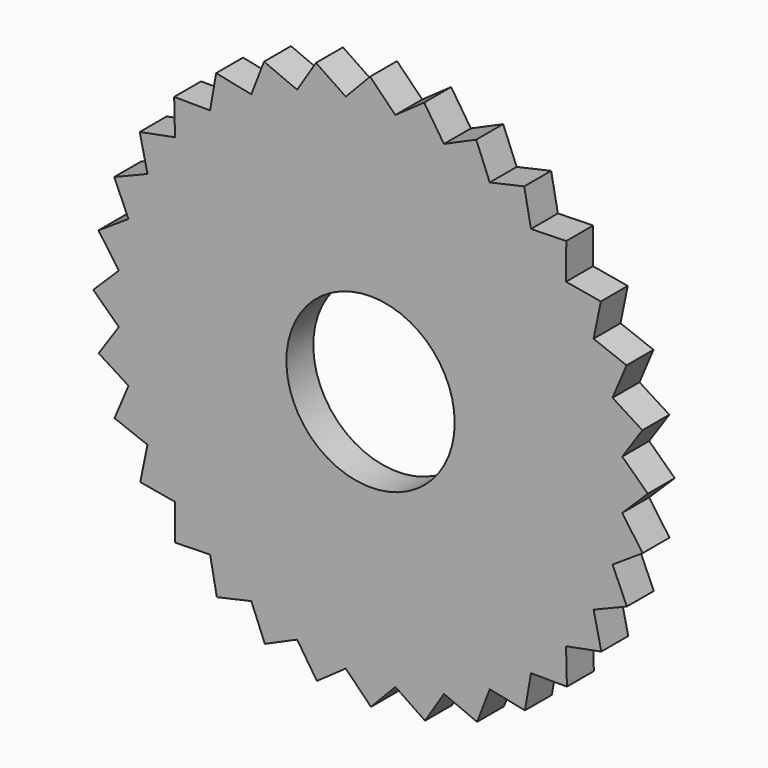
from build123d import *

# Parameters (mm, degrees)
F1_DEPTH = 5.08
F2_DEPTH = 5.08
F3_DEPTH = 5.08


with BuildPart() as f1:
    # F0 (on Front) → F1 (new body, symmetric)
    with BuildSketch(Plane.XZ):
        with BuildLine():
            ThreePointArc((75.8478085303, 7.3177825298), (76.1119012048, 3.6631263964), (76.2, 0))
            ThreePointArc((76.2, 0), (76.1119012048, -3.6631263964), (75.8478085303, -7.3177825298))
            Line((75.8478085303, -7.3177825298), (75.9612060886, -7.4788283967))
            Line((75.9612060886, -7.4788283967), (83.6803820326, 0.1329535853))
            Line((83.6803820326, 0.1329535853), (75.9606798536, 7.4841713504))
            Line((75.9606798536, 7.4841713504), (75.8478085303, 7.3177825298))
        make_face()
        with BuildLine():
            ThreePointArc((75.8180427075, 7.62), (75.8330761724, 7.4689060931), (75.8478085303, 7.3177825298))
            Line((75.8478085303, 7.3177825298), (75.9606798536, 7.4841713504))
            Line((75.9606798536, 7.4841713504), (75.8180427075, 7.62))
        make_face()
        with BuildLine():
            Line((75.9612060886, -7.4788283967), (75.8478085303, -7.3177825298))
            ThreePointArc((75.8478085303, -7.3177825298), (75.8330761724, -7.4689060931), (75.8180427075, -7.62))
            Line((75.8180427075, -7.62), (75.9612060886, -7.4788283967))
        make_face()
        with BuildLine():
            ThreePointArc((72.9627856072, 21.9743467808), (74.7358383667, 14.8658825376), (75.8180427075, 7.62))
            Line((75.8180427075, 7.62), (75.9606798536, 7.4841713504))
            Line((75.9606798536, 7.4841713504), (82.0465489983, 16.4556315966))
            Line((82.0465489983, 16.4556315966), (73.041027291, 22.1595585897))
            Line((73.041027291, 22.1595585897), (72.9627856072, 21.9743467808))
        make_face()
        with BuildLine():
            Line((75.9612060886, -7.4788283967), (75.8180427075, -7.62))
            ThreePointArc((75.8180427075, -7.62), (74.7358383667, -14.8658825376), (72.9627856072, -21.9743467808))
            Line((72.9627856072, -21.9743467808), (73.0425857732, -22.1544209627))
            Line((73.0425857732, -22.1544209627), (82.0984249139, -16.1948337577))
            Line((82.0984249139, -16.1948337577), (75.9612060886, -7.4788283967))
        make_face()
        with BuildLine():
            ThreePointArc((72.8746320228, 22.2649502031), (72.9188535828, 22.1196924068), (72.9627856072, 21.9743467808))
            Line((72.9627856072, 21.9743467808), (73.041027291, 22.1595585897))
            Line((73.041027291, 22.1595585897), (72.8746320228, 22.2649502031))
        make_face()
        with BuildLine():
            Line((73.0425857732, -22.1544209627), (72.9627856072, -21.9743467808))
            ThreePointArc((72.9627856072, -21.9743467808), (72.9188535828, -22.1196924068), (72.8746320228, -22.2649502031))
            Line((72.8746320228, -22.2649502031), (73.0425857732, -22.1544209627))
        make_face()
        with BuildLine():
            ThreePointArc((67.2738437512, 35.7864492084), (70.3996203774, 29.1604775462), (72.8746320228, 22.2649502031))
            Line((72.8746320228, 22.2649502031), (73.041027291, 22.1595585897))
            Line((73.041027291, 22.1595585897), (77.2597130983, 32.1459289141))
            Line((77.2597130983, 32.1459289141), (67.3144490116, 35.9833664196))
            Line((67.3144490116, 35.9833664196), (67.2738437512, 35.7864492084))
        make_face()
        with BuildLine():
            Line((73.0425857732, -22.1544209627), (72.8746320228, -22.2649502031))
            ThreePointArc((72.8746320228, -22.2649502031), (70.3996203774, -29.1604775462), (67.2738437512, -35.7864492084))
            Line((67.2738437512, -35.7864492084), (67.3169798492, -35.9786315554))
            Line((67.3169798492, -35.9786315554), (77.361471367, -31.9002627216))
            Line((77.361471367, -31.9002627216), (73.0425857732, -22.1544209627))
        make_face()
        with BuildLine():
            ThreePointArc((67.1306900979, 36.0542708563), (67.2024003433, 35.9204313461), (67.2738437512, 35.7864492084))
            Line((67.2738437512, 35.7864492084), (67.3144490116, 35.9833664196))
            Line((67.3144490116, 35.9833664196), (67.1306900979, 36.0542708563))
        make_face()
        with BuildLine():
            Line((67.3169798492, -35.9786315554), (67.2738437512, -35.7864492084))
            ThreePointArc((67.2738437512, -35.7864492084), (67.2024003433, -35.9204313461), (67.1306900979, -36.0542708563))
            Line((67.1306900979, -36.0542708563), (67.3169798492, -35.9786315554))
        make_face()
        with BuildLine():
            ThreePointArc((58.9996058074, 48.2232984621), (63.3579844575, 42.3344517561), (67.1306900979, 36.0542708563))
            Line((67.1306900979, 36.0542708563), (67.3144490116, 35.9833664196))
            Line((67.3144490116, 35.9833664196), (69.5038297516, 46.6008762111))
            Line((69.5038297516, 46.6008762111), (59.001014207, 48.4243536577))
            Line((59.001014207, 48.4243536577), (58.9996058074, 48.2232984621))
        make_face()
        with BuildLine():
            Line((67.3169798492, -35.9786315554), (67.1306900979, -36.0542708563))
            ThreePointArc((67.1306900979, -36.0542708563), (63.3579844575, -42.3344517561), (58.9996058074, -48.2232984621))
            Line((58.9996058074, -48.2232984621), (59.0044201415, -48.4202035145))
            Line((59.0044201415, -48.4202035145), (69.6515598604, -46.379782479))
            Line((69.6515598604, -46.379782479), (67.3169798492, -35.9786315554))
        make_face()
        with BuildLine():
            ThreePointArc((58.8069534, 48.4580460999), (58.9033965462, 48.3407682533), (58.9996058074, 48.2232984621))
            Line((58.9996058074, 48.2232984621), (59.001014207, 48.4243536577))
            Line((59.001014207, 48.4243536577), (58.8069534, 48.4580460999))
        make_face()
        with BuildLine():
            Line((59.0044201415, -48.4202035145), (58.9996058074, -48.2232984621))
            ThreePointArc((58.9996058074, -48.2232984621), (58.9033965462, -48.3407682533), (58.8069534, -48.4580460999))
            Line((58.8069534, -48.4580460999), (59.0044201415, -48.4202035145))
        make_face()
        with BuildLine():
            ThreePointArc((48.4580460999, 58.8069534), (53.8815367264, 53.8815367264), (58.8069534, 48.4580460999))
            Line((58.8069534, 48.4580460999), (59.001014207, 48.4243536577))
            Line((59.001014207, 48.4243536577), (59.0769532058, 59.2649779693))
            Line((59.0769532058, 59.2649779693), (48.4202035145, 59.0044201415))
            Line((48.4202035145, 59.0044201415), (48.4580460999, 58.8069534))
        make_face()
        with BuildLine():
            Line((59.0044201415, -48.4202035145), (58.8069534, -48.4580460999))
            ThreePointArc((58.8069534, -48.4580460999), (53.8815367264, -53.8815367264), (48.4580460999, -58.8069534))
            Line((48.4580460999, -58.8069534), (48.4243536577, -59.001014207))
            Line((48.4243536577, -59.001014207), (59.2649779693, -59.0769532058))
            Line((59.2649779693, -59.0769532058), (59.0044201415, -48.4202035145))
        make_face()
        with BuildLine():
            ThreePointArc((48.2232984621, 58.9996058074), (48.3407682533, 58.9033965462), (48.4580460999, 58.8069534))
            Line((48.4580460999, 58.8069534), (48.4202035145, 59.0044201415))
            Line((48.4202035145, 59.0044201415), (48.2232984621, 58.9996058074))
        make_face()
        with BuildLine():
            Line((48.4243536577, -59.001014207), (48.4580460999, -58.8069534))
            ThreePointArc((48.4580460999, -58.8069534), (48.3407682533, -58.9033965462), (48.2232984621, -58.9996058074))
            Line((48.2232984621, -58.9996058074), (48.4243536577, -59.001014207))
        make_face()
        with BuildLine():
            ThreePointArc((36.0542708563, 67.1306900979), (42.3344517561, 63.3579844575), (48.2232984621, 58.9996058074))
            Line((48.2232984621, 58.9996058074), (48.4202035145, 59.0044201415))
            Line((48.4202035145, 59.0044201415), (46.379782479, 69.6515598604))
            Line((46.379782479, 69.6515598604), (35.9786315554, 67.3169798492))
            Line((35.9786315554, 67.3169798492), (36.0542708563, 67.1306900979))
        make_face()
        with BuildLine():
            Line((48.4243536577, -59.001014207), (48.2232984621, -58.9996058074))
            ThreePointArc((48.2232984621, -58.9996058074), (42.3344517561, -63.3579844575), (36.0542708563, -67.1306900979))
            Line((36.0542708563, -67.1306900979), (35.9833664196, -67.3144490116))
            Line((35.9833664196, -67.3144490116), (46.6008762111, -69.5038297516))
            Line((46.6008762111, -69.5038297516), (48.4243536577, -59.001014207))
        make_face()
        with BuildLine():
            ThreePointArc((35.7864492084, 67.2738437512), (35.9204313461, 67.2024003433), (36.0542708563, 67.1306900979))
            Line((36.0542708563, 67.1306900979), (35.9786315554, 67.3169798492))
            Line((35.9786315554, 67.3169798492), (35.7864492084, 67.2738437512))
        make_face()
        with BuildLine():
            Line((35.9833664196, -67.3144490116), (36.0542708563, -67.1306900979))
            ThreePointArc((36.0542708563, -67.1306900979), (35.9204313461, -67.2024003433), (35.7864492084, -67.2738437512))
            Line((35.7864492084, -67.2738437512), (35.9833664196, -67.3144490116))
        make_face()
        with BuildLine():
            ThreePointArc((22.2649502031, 72.8746320228), (29.1604775462, 70.3996203774), (35.7864492084, 67.2738437512))
            Line((35.7864492084, 67.2738437512), (35.9786315554, 67.3169798492))
            Line((35.9786315554, 67.3169798492), (31.9002627216, 77.361471367))
            Line((31.9002627216, 77.361471367), (22.1544209627, 73.0425857732))
            Line((22.1544209627, 73.0425857732), (22.2649502031, 72.8746320228))
        make_face()
        with BuildLine():
            Line((35.9833664196, -67.3144490116), (35.7864492084, -67.2738437512))
            ThreePointArc((35.7864492084, -67.2738437512), (29.1604775462, -70.3996203774), (22.2649502031, -72.8746320228))
            Line((22.2649502031, -72.8746320228), (22.1595585897, -73.041027291))
            Line((22.1595585897, -73.041027291), (32.1459289141, -77.2597130983))
            Line((32.1459289141, -77.2597130983), (35.9833664196, -67.3144490116))
        make_face()
        with BuildLine():
            ThreePointArc((21.9743467808, 72.9627856072), (22.1196924068, 72.9188535828), (22.2649502031, 72.8746320228))
            Line((22.2649502031, 72.8746320228), (22.1544209627, 73.0425857732))
            Line((22.1544209627, 73.0425857732), (21.9743467808, 72.9627856072))
        make_face()
        with BuildLine():
            Line((22.1595585897, -73.041027291), (22.2649502031, -72.8746320228))
            ThreePointArc((22.2649502031, -72.8746320228), (22.1196924068, -72.9188535828), (21.9743467808, -72.9627856072))
            Line((21.9743467808, -72.9627856072), (22.1595585897, -73.041027291))
        make_face()
        with BuildLine():
            ThreePointArc((7.62, 75.8180427075), (14.8658825376, 74.7358383667), (21.9743467808, 72.9627856072))
            Line((21.9743467808, 72.9627856072), (22.1544209627, 73.0425857732))
            Line((22.1544209627, 73.0425857732), (16.1948337577, 82.0984249139))
            Line((16.1948337577, 82.0984249139), (7.4788283967, 75.9612060886))
            Line((7.4788283967, 75.9612060886), (7.62, 75.8180427075))
        make_face()
        with BuildLine():
            Line((22.1595585897, -73.041027291), (21.9743467808, -72.9627856072))
            ThreePointArc((21.9743467808, -72.9627856072), (14.8658825376, -74.7358383667), (7.62, -75.8180427075))
            Line((7.62, -75.8180427075), (7.4841713504, -75.9606798536))
            Line((7.4841713504, -75.9606798536), (16.4556315966, -82.0465489983))
            Line((16.4556315966, -82.0465489983), (22.1595585897, -73.041027291))
        make_face()
        with BuildLine():
            ThreePointArc((7.3177825298, 75.8478085303), (7.4689060931, 75.8330761724), (7.62, 75.8180427075))
            Line((7.62, 75.8180427075), (7.4788283967, 75.9612060886))
            Line((7.4788283967, 75.9612060886), (7.3177825298, 75.8478085303))
        make_face()
        with BuildLine():
            Line((7.4841713504, -75.9606798536), (7.62, -75.8180427075))
            ThreePointArc((7.62, -75.8180427075), (7.4689060931, -75.8330761724), (7.3177825298, -75.8478085303))
            Line((7.3177825298, -75.8478085303), (7.4841713504, -75.9606798536))
        make_face()
        with BuildLine():
            ThreePointArc((0, 76.2), (3.6631263964, 76.1119012048), (7.3177825298, 75.8478085303))
            Line((7.3177825298, 75.8478085303), (7.4788283967, 75.9612060886))
            Line((7.4788283967, 75.9612060886), (-0.1329535853, 83.6803820326))
            Line((-0.1329535853, 83.6803820326), (-7.4841713504, 75.9606798536))
            Line((-7.4841713504, 75.9606798536), (-7.3177825298, 75.8478085303))
            ThreePointArc((-7.3177825298, 75.8478085303), (-3.6631263964, 76.1119012048), (0, 76.2))
        make_face()
        with BuildLine():
            Line((7.4841713504, -75.9606798536), (7.3177825298, -75.8478085303))
            ThreePointArc((7.3177825298, -75.8478085303), (0, -76.2), (-7.3177825298, -75.8478085303))
            Line((-7.3177825298, -75.8478085303), (-7.4788283967, -75.9612060886))
            Line((-7.4788283967, -75.9612060886), (0.1329535853, -83.6803820326))
            Line((0.1329535853, -83.6803820326), (7.4841713504, -75.9606798536))
        make_face()
        with BuildLine():
            Line((-7.4788283967, -75.9612060886), (-7.3177825298, -75.8478085303))
            ThreePointArc((-7.3177825298, -75.8478085303), (-7.4689060931, -75.8330761724), (-7.62, -75.8180427075))
            Line((-7.62, -75.8180427075), (-7.4788283967, -75.9612060886))
        make_face()
        with BuildLine():
            ThreePointArc((-7.62, 75.8180427075), (-7.4689060931, 75.8330761724), (-7.3177825298, 75.8478085303))
            Line((-7.3177825298, 75.8478085303), (-7.4841713504, 75.9606798536))
            Line((-7.4841713504, 75.9606798536), (-7.62, 75.8180427075))
        make_face()
        with BuildLine():
            Line((-7.62, 75.8180427075), (-7.4841713504, 75.9606798536))
            Line((-7.4841713504, 75.9606798536), (-16.4556315966, 82.0465489983))
            Line((-16.4556315966, 82.0465489983), (-22.1595585897, 73.041027291))
            Line((-22.1595585897, 73.041027291), (-21.9743467808, 72.9627856072))
            ThreePointArc((-21.9743467808, 72.9627856072), (-14.8658825376, 74.7358383667), (-7.62, 75.8180427075))
        make_face()
        with BuildLine():
            Line((-7.4788283967, -75.9612060886), (-7.62, -75.8180427075))
            ThreePointArc((-7.62, -75.8180427075), (-14.8658825376, -74.7358383667), (-21.9743467808, -72.9627856072))
            Line((-21.9743467808, -72.9627856072), (-22.1544209627, -73.0425857732))
            Line((-22.1544209627, -73.0425857732), (-16.1948337577, -82.0984249139))
            Line((-16.1948337577, -82.0984249139), (-7.4788283967, -75.9612060886))
        make_face()
        with BuildLine():
            Line((-22.1544209627, -73.0425857732), (-21.9743467808, -72.9627856072))
            ThreePointArc((-21.9743467808, -72.9627856072), (-22.1196924068, -72.9188535828), (-22.2649502031, -72.8746320228))
            Line((-22.2649502031, -72.8746320228), (-22.1544209627, -73.0425857732))
        make_face()
        with BuildLine():
            ThreePointArc((-22.2649502031, 72.8746320228), (-22.1196924068, 72.9188535828), (-21.9743467808, 72.9627856072))
            Line((-21.9743467808, 72.9627856072), (-22.1595585897, 73.041027291))
            Line((-22.1595585897, 73.041027291), (-22.2649502031, 72.8746320228))
        make_face()
        with BuildLine():
            Line((-22.2649502031, 72.8746320228), (-22.1595585897, 73.041027291))
            Line((-22.1595585897, 73.041027291), (-32.1459289141, 77.2597130983))
            Line((-32.1459289141, 77.2597130983), (-35.9833664196, 67.3144490116))
            Line((-35.9833664196, 67.3144490116), (-35.7864492084, 67.2738437512))
            ThreePointArc((-35.7864492084, 67.2738437512), (-29.1604775462, 70.3996203774), (-22.2649502031, 72.8746320228))
        make_face()
        with BuildLine():
            Line((-22.1544209627, -73.0425857732), (-22.2649502031, -72.8746320228))
            ThreePointArc((-22.2649502031, -72.8746320228), (-29.1604775462, -70.3996203774), (-35.7864492084, -67.2738437512))
            Line((-35.7864492084, -67.2738437512), (-35.9786315554, -67.3169798492))
            Line((-35.9786315554, -67.3169798492), (-31.9002627216, -77.361471367))
            Line((-31.9002627216, -77.361471367), (-22.1544209627, -73.0425857732))
        make_face()
        with BuildLine():
            Line((-35.9786315554, -67.3169798492), (-35.7864492084, -67.2738437512))
            ThreePointArc((-35.7864492084, -67.2738437512), (-35.9204313461, -67.2024003433), (-36.0542708563, -67.1306900979))
            Line((-36.0542708563, -67.1306900979), (-35.9786315554, -67.3169798492))
        make_face()
        with BuildLine():
            ThreePointArc((-36.0542708563, 67.1306900979), (-35.9204313461, 67.2024003433), (-35.7864492084, 67.2738437512))
            Line((-35.7864492084, 67.2738437512), (-35.9833664196, 67.3144490116))
            Line((-35.9833664196, 67.3144490116), (-36.0542708563, 67.1306900979))
        make_face()
        with BuildLine():
            Line((-36.0542708563, 67.1306900979), (-35.9833664196, 67.3144490116))
            Line((-35.9833664196, 67.3144490116), (-46.6008762111, 69.5038297516))
            Line((-46.6008762111, 69.5038297516), (-48.4243536577, 59.001014207))
            Line((-48.4243536577, 59.001014207), (-48.2232984621, 58.9996058074))
            ThreePointArc((-48.2232984621, 58.9996058074), (-42.3344517561, 63.3579844575), (-36.0542708563, 67.1306900979))
        make_face()
        with BuildLine():
            Line((-35.9786315554, -67.3169798492), (-36.0542708563, -67.1306900979))
            ThreePointArc((-36.0542708563, -67.1306900979), (-42.3344517561, -63.3579844575), (-48.2232984621, -58.9996058074))
            Line((-48.2232984621, -58.9996058074), (-48.4202035145, -59.0044201415))
            Line((-48.4202035145, -59.0044201415), (-46.379782479, -69.6515598604))
            Line((-46.379782479, -69.6515598604), (-35.9786315554, -67.3169798492))
        make_face()
        with BuildLine():
            Line((-48.4202035145, -59.0044201415), (-48.2232984621, -58.9996058074))
            ThreePointArc((-48.2232984621, -58.9996058074), (-48.3407682533, -58.9033965462), (-48.4580460999, -58.8069534))
            Line((-48.4580460999, -58.8069534), (-48.4202035145, -59.0044201415))
        make_face()
        with BuildLine():
            ThreePointArc((-48.4580460999, 58.8069534), (-48.3407682533, 58.9033965462), (-48.2232984621, 58.9996058074))
            Line((-48.2232984621, 58.9996058074), (-48.4243536577, 59.001014207))
            Line((-48.4243536577, 59.001014207), (-48.4580460999, 58.8069534))
        make_face()
        with BuildLine():
            Line((-48.4580460999, 58.8069534), (-48.4243536577, 59.001014207))
            Line((-48.4243536577, 59.001014207), (-59.2649779693, 59.0769532058))
            Line((-59.2649779693, 59.0769532058), (-59.0044201415, 48.4202035145))
            Line((-59.0044201415, 48.4202035145), (-58.8069534, 48.4580460999))
            ThreePointArc((-58.8069534, 48.4580460999), (-53.8815367264, 53.8815367264), (-48.4580460999, 58.8069534))
        make_face()
        with BuildLine():
            Line((-48.4202035145, -59.0044201415), (-48.4580460999, -58.8069534))
            ThreePointArc((-48.4580460999, -58.8069534), (-53.8815367264, -53.8815367264), (-58.8069534, -48.4580460999))
            Line((-58.8069534, -48.4580460999), (-59.001014207, -48.4243536577))
            Line((-59.001014207, -48.4243536577), (-59.0769532058, -59.2649779693))
            Line((-59.0769532058, -59.2649779693), (-48.4202035145, -59.0044201415))
        make_face()
        with BuildLine():
            Line((-59.001014207, -48.4243536577), (-58.8069534, -48.4580460999))
            ThreePointArc((-58.8069534, -48.4580460999), (-58.9033965462, -48.3407682533), (-58.9996058074, -48.2232984621))
            Line((-58.9996058074, -48.2232984621), (-59.001014207, -48.4243536577))
        make_face()
        with BuildLine():
            ThreePointArc((-58.9996058074, 48.2232984621), (-58.9033965462, 48.3407682533), (-58.8069534, 48.4580460999))
            Line((-58.8069534, 48.4580460999), (-59.0044201415, 48.4202035145))
            Line((-59.0044201415, 48.4202035145), (-58.9996058074, 48.2232984621))
        make_face()
        with BuildLine():
            Line((-58.9996058074, 48.2232984621), (-59.0044201415, 48.4202035145))
            Line((-59.0044201415, 48.4202035145), (-69.6515598604, 46.379782479))
            Line((-69.6515598604, 46.379782479), (-67.3169798492, 35.9786315554))
            Line((-67.3169798492, 35.9786315554), (-67.1306900979, 36.0542708563))
            ThreePointArc((-67.1306900979, 36.0542708563), (-63.3579844575, 42.3344517561), (-58.9996058074, 48.2232984621))
        make_face()
        with BuildLine():
            Line((-59.001014207, -48.4243536577), (-58.9996058074, -48.2232984621))
            ThreePointArc((-58.9996058074, -48.2232984621), (-63.3579844575, -42.3344517561), (-67.1306900979, -36.0542708563))
            Line((-67.1306900979, -36.0542708563), (-67.3144490116, -35.9833664196))
            Line((-67.3144490116, -35.9833664196), (-69.5038297516, -46.6008762111))
            Line((-69.5038297516, -46.6008762111), (-59.001014207, -48.4243536577))
        make_face()
        with BuildLine():
            Line((-67.3144490116, -35.9833664196), (-67.1306900979, -36.0542708563))
            ThreePointArc((-67.1306900979, -36.0542708563), (-67.2024003433, -35.9204313461), (-67.2738437512, -35.7864492084))
            Line((-67.2738437512, -35.7864492084), (-67.3144490116, -35.9833664196))
        make_face()
        with BuildLine():
            ThreePointArc((-67.2738437512, 35.7864492084), (-67.2024003433, 35.9204313461), (-67.1306900979, 36.0542708563))
            Line((-67.1306900979, 36.0542708563), (-67.3169798492, 35.9786315554))
            Line((-67.3169798492, 35.9786315554), (-67.2738437512, 35.7864492084))
        make_face()
        with BuildLine():
            Line((-67.2738437512, 35.7864492084), (-67.3169798492, 35.9786315554))
            Line((-67.3169798492, 35.9786315554), (-77.361471367, 31.9002627216))
            Line((-77.361471367, 31.9002627216), (-73.0425857732, 22.1544209627))
            Line((-73.0425857732, 22.1544209627), (-72.8746320228, 22.2649502031))
            ThreePointArc((-72.8746320228, 22.2649502031), (-70.3996203774, 29.1604775462), (-67.2738437512, 35.7864492084))
        make_face()
        with BuildLine():
            Line((-67.3144490116, -35.9833664196), (-67.2738437512, -35.7864492084))
            ThreePointArc((-67.2738437512, -35.7864492084), (-70.3996203774, -29.1604775462), (-72.8746320228, -22.2649502031))
            Line((-72.8746320228, -22.2649502031), (-73.041027291, -22.1595585897))
            Line((-73.041027291, -22.1595585897), (-77.2597130983, -32.1459289141))
            Line((-77.2597130983, -32.1459289141), (-67.3144490116, -35.9833664196))
        make_face()
        with BuildLine():
            Line((-73.041027291, -22.1595585897), (-72.8746320228, -22.2649502031))
            ThreePointArc((-72.8746320228, -22.2649502031), (-72.9188535828, -22.1196924068), (-72.9627856072, -21.9743467808))
            Line((-72.9627856072, -21.9743467808), (-73.041027291, -22.1595585897))
        make_face()
        with BuildLine():
            ThreePointArc((-72.9627856072, 21.9743467808), (-72.9188535828, 22.1196924068), (-72.8746320228, 22.2649502031))
            Line((-72.8746320228, 22.2649502031), (-73.0425857732, 22.1544209627))
            Line((-73.0425857732, 22.1544209627), (-72.9627856072, 21.9743467808))
        make_face()
        with BuildLine():
            Line((-72.9627856072, 21.9743467808), (-73.0425857732, 22.1544209627))
            Line((-73.0425857732, 22.1544209627), (-82.0984249139, 16.1948337577))
            Line((-82.0984249139, 16.1948337577), (-75.9612060886, 7.4788283967))
            Line((-75.9612060886, 7.4788283967), (-75.8180427075, 7.62))
            ThreePointArc((-75.8180427075, 7.62), (-74.7358383667, 14.8658825376), (-72.9627856072, 21.9743467808))
        make_face()
        with BuildLine():
            Line((-73.041027291, -22.1595585897), (-72.9627856072, -21.9743467808))
            ThreePointArc((-72.9627856072, -21.9743467808), (-74.7358383667, -14.8658825376), (-75.8180427075, -7.62))
            Line((-75.8180427075, -7.62), (-75.9606798536, -7.4841713504))
            Line((-75.9606798536, -7.4841713504), (-82.0465489983, -16.4556315966))
            Line((-82.0465489983, -16.4556315966), (-73.041027291, -22.1595585897))
        make_face()
        with BuildLine():
            Line((-75.9606798536, -7.4841713504), (-75.8180427075, -7.62))
            ThreePointArc((-75.8180427075, -7.62), (-75.8330761724, -7.4689060931), (-75.8478085303, -7.3177825298))
            Line((-75.8478085303, -7.3177825298), (-75.9606798536, -7.4841713504))
        make_face()
        with BuildLine():
            ThreePointArc((-75.8478085303, 7.3177825298), (-75.8330761724, 7.4689060931), (-75.8180427075, 7.62))
            Line((-75.8180427075, 7.62), (-75.9612060886, 7.4788283967))
            Line((-75.9612060886, 7.4788283967), (-75.8478085303, 7.3177825298))
        make_face()
        with BuildLine():
            Line((-75.8478085303, 7.3177825298), (-75.9612060886, 7.4788283967))
            Line((-75.9612060886, 7.4788283967), (-83.6803820326, -0.1329535853))
            Line((-83.6803820326, -0.1329535853), (-75.9606798536, -7.4841713504))
            Line((-75.9606798536, -7.4841713504), (-75.8478085303, -7.3177825298))
            ThreePointArc((-75.8478085303, -7.3177825298), (-76.2, 0), (-75.8478085303, 7.3177825298))
        make_face()
    extrude(amount=F1_DEPTH, both=True)

    # F0 (on Front) → F2 (join, symmetric)
    with BuildSketch(Plane.XZ):
        with BuildLine():
            ThreePointArc((75.8478085303, -7.3177825298), (76.1119012048, -3.6631263964), (76.2, 0))
            ThreePointArc((76.2, 0), (76.1119012048, 3.6631263964), (75.8478085303, 7.3177825298))
            ThreePointArc((75.8478085303, 7.3177825298), (75.8330761724, 7.4689060931), (75.8180427075, 7.62))
            ThreePointArc((75.8180427075, 7.62), (74.7358383667, 14.8658825376), (72.9627856072, 21.9743467808))
            ThreePointArc((72.9627856072, 21.9743467808), (72.9188535828, 22.1196924068), (72.8746320228, 22.2649502031))
            ThreePointArc((72.8746320228, 22.2649502031), (70.3996203774, 29.1604775462), (67.2738437512, 35.7864492084))
            ThreePointArc((67.2738437512, 35.7864492084), (67.2024003433, 35.9204313461), (67.1306900979, 36.0542708563))
            ThreePointArc((67.1306900979, 36.0542708563), (63.3579844575, 42.3344517561), (58.9996058074, 48.2232984621))
            ThreePointArc((58.9996058074, 48.2232984621), (58.9033965462, 48.3407682533), (58.8069534, 48.4580460999))
            ThreePointArc((58.8069534, 48.4580460999), (53.8815367264, 53.8815367264), (48.4580460999, 58.8069534))
            ThreePointArc((48.4580460999, 58.8069534), (48.3407682533, 58.9033965462), (48.2232984621, 58.9996058074))
            ThreePointArc((48.2232984621, 58.9996058074), (42.3344517561, 63.3579844575), (36.0542708563, 67.1306900979))
            ThreePointArc((36.0542708563, 67.1306900979), (35.9204313461, 67.2024003433), (35.7864492084, 67.2738437512))
            ThreePointArc((35.7864492084, 67.2738437512), (29.1604775462, 70.3996203774), (22.2649502031, 72.8746320228))
            ThreePointArc((22.2649502031, 72.8746320228), (22.1196924068, 72.9188535828), (21.9743467808, 72.9627856072))
            ThreePointArc((21.9743467808, 72.9627856072), (14.8658825376, 74.7358383667), (7.62, 75.8180427075))
            ThreePointArc((7.62, 75.8180427075), (7.4689060931, 75.8330761724), (7.3177825298, 75.8478085303))
            ThreePointArc((7.3177825298, 75.8478085303), (3.6631263964, 76.1119012048), (0, 76.2))
            ThreePointArc((0, 76.2), (-3.6631263964, 76.1119012048), (-7.3177825298, 75.8478085303))
            ThreePointArc((-7.3177825298, 75.8478085303), (-7.4689060931, 75.8330761724), (-7.62, 75.8180427075))
            ThreePointArc((-7.62, 75.8180427075), (-14.8658825376, 74.7358383667), (-21.9743467808, 72.9627856072))
            ThreePointArc((-21.9743467808, 72.9627856072), (-22.1196924068, 72.9188535828), (-22.2649502031, 72.8746320228))
            ThreePointArc((-22.2649502031, 72.8746320228), (-29.1604775462, 70.3996203774), (-35.7864492084, 67.2738437512))
            ThreePointArc((-35.7864492084, 67.2738437512), (-35.9204313461, 67.2024003433), (-36.0542708563, 67.1306900979))
            ThreePointArc((-36.0542708563, 67.1306900979), (-42.3344517561, 63.3579844575), (-48.2232984621, 58.9996058074))
            ThreePointArc((-48.2232984621, 58.9996058074), (-48.3407682533, 58.9033965462), (-48.4580460999, 58.8069534))
            ThreePointArc((-48.4580460999, 58.8069534), (-53.8815367264, 53.8815367264), (-58.8069534, 48.4580460999))
            ThreePointArc((-58.8069534, 48.4580460999), (-58.9033965462, 48.3407682533), (-58.9996058074, 48.2232984621))
            ThreePointArc((-58.9996058074, 48.2232984621), (-63.3579844575, 42.3344517561), (-67.1306900979, 36.0542708563))
            ThreePointArc((-67.1306900979, 36.0542708563), (-67.2024003433, 35.9204313461), (-67.2738437512, 35.7864492084))
            ThreePointArc((-67.2738437512, 35.7864492084), (-70.3996203774, 29.1604775462), (-72.8746320228, 22.2649502031))
            ThreePointArc((-72.8746320228, 22.2649502031), (-72.9188535828, 22.1196924068), (-72.9627856072, 21.9743467808))
            ThreePointArc((-72.9627856072, 21.9743467808), (-74.7358383667, 14.8658825376), (-75.8180427075, 7.62))
            ThreePointArc((-75.8180427075, 7.62), (-75.8330761724, 7.4689060931), (-75.8478085303, 7.3177825298))
            ThreePointArc((-75.8478085303, 7.3177825298), (-76.2, 0), (-75.8478085303, -7.3177825298))
            ThreePointArc((-75.8478085303, -7.3177825298), (-75.8330761724, -7.4689060931), (-75.8180427075, -7.62))
            ThreePointArc((-75.8180427075, -7.62), (-74.7358383667, -14.8658825376), (-72.9627856072, -21.9743467808))
            ThreePointArc((-72.9627856072, -21.9743467808), (-72.9188535828, -22.1196924068), (-72.8746320228, -22.2649502031))
            ThreePointArc((-72.8746320228, -22.2649502031), (-70.3996203774, -29.1604775462), (-67.2738437512, -35.7864492084))
            ThreePointArc((-67.2738437512, -35.7864492084), (-67.2024003433, -35.9204313461), (-67.1306900979, -36.0542708563))
            ThreePointArc((-67.1306900979, -36.0542708563), (-63.3579844575, -42.3344517561), (-58.9996058074, -48.2232984621))
            ThreePointArc((-58.9996058074, -48.2232984621), (-58.9033965462, -48.3407682533), (-58.8069534, -48.4580460999))
            ThreePointArc((-58.8069534, -48.4580460999), (-53.8815367264, -53.8815367264), (-48.4580460999, -58.8069534))
            ThreePointArc((-48.4580460999, -58.8069534), (-48.3407682533, -58.9033965462), (-48.2232984621, -58.9996058074))
            ThreePointArc((-48.2232984621, -58.9996058074), (-42.3344517561, -63.3579844575), (-36.0542708563, -67.1306900979))
            ThreePointArc((-36.0542708563, -67.1306900979), (-35.9204313461, -67.2024003433), (-35.7864492084, -67.2738437512))
            ThreePointArc((-35.7864492084, -67.2738437512), (-29.1604775462, -70.3996203774), (-22.2649502031, -72.8746320228))
            ThreePointArc((-22.2649502031, -72.8746320228), (-22.1196924068, -72.9188535828), (-21.9743467808, -72.9627856072))
            ThreePointArc((-21.9743467808, -72.9627856072), (-14.8658825376, -74.7358383667), (-7.62, -75.8180427075))
            ThreePointArc((-7.62, -75.8180427075), (-7.4689060931, -75.8330761724), (-7.3177825298, -75.8478085303))
            ThreePointArc((-7.3177825298, -75.8478085303), (0, -76.2), (7.3177825298, -75.8478085303))
            ThreePointArc((7.3177825298, -75.8478085303), (7.4689060931, -75.8330761724), (7.62, -75.8180427075))
            ThreePointArc((7.62, -75.8180427075), (14.8658825376, -74.7358383667), (21.9743467808, -72.9627856072))
            ThreePointArc((21.9743467808, -72.9627856072), (22.1196924068, -72.9188535828), (22.2649502031, -72.8746320228))
            ThreePointArc((22.2649502031, -72.8746320228), (29.1604775462, -70.3996203774), (35.7864492084, -67.2738437512))
            ThreePointArc((35.7864492084, -67.2738437512), (35.9204313461, -67.2024003433), (36.0542708563, -67.1306900979))
            ThreePointArc((36.0542708563, -67.1306900979), (42.3344517561, -63.3579844575), (48.2232984621, -58.9996058074))
            ThreePointArc((48.2232984621, -58.9996058074), (48.3407682533, -58.9033965462), (48.4580460999, -58.8069534))
            ThreePointArc((48.4580460999, -58.8069534), (53.8815367264, -53.8815367264), (58.8069534, -48.4580460999))
            ThreePointArc((58.8069534, -48.4580460999), (58.9033965462, -48.3407682533), (58.9996058074, -48.2232984621))
            ThreePointArc((58.9996058074, -48.2232984621), (63.3579844575, -42.3344517561), (67.1306900979, -36.0542708563))
            ThreePointArc((67.1306900979, -36.0542708563), (67.2024003433, -35.9204313461), (67.2738437512, -35.7864492084))
            ThreePointArc((67.2738437512, -35.7864492084), (70.3996203774, -29.1604775462), (72.8746320228, -22.2649502031))
            ThreePointArc((72.8746320228, -22.2649502031), (72.9188535828, -22.1196924068), (72.9627856072, -21.9743467808))
            ThreePointArc((72.9627856072, -21.9743467808), (74.7358383667, -14.8658825376), (75.8180427075, -7.62))
            ThreePointArc((75.8180427075, -7.62), (75.8330761724, -7.4689060931), (75.8478085303, -7.3177825298))
        make_face()
        with BuildLine():
            ThreePointArc((25.4, 0), (-17.9605122421, -17.9605122421), (0, 25.4))
            ThreePointArc((0, 25.4), (17.9605122421, 17.9605122421), (25.4, 0))
        make_face(mode=Mode.SUBTRACT)
    extrude(amount=F2_DEPTH, both=True)

    # F0 (on Front) → F3 (join, symmetric)
    with BuildSketch(Plane.XZ):
        with BuildLine():
            ThreePointArc((75.8478085303, -7.3177825298), (76.1119012048, -3.6631263964), (76.2, 0))
            ThreePointArc((76.2, 0), (76.1119012048, 3.6631263964), (75.8478085303, 7.3177825298))
            ThreePointArc((75.8478085303, 7.3177825298), (75.8330761724, 7.4689060931), (75.8180427075, 7.62))
            ThreePointArc((75.8180427075, 7.62), (74.7358383667, 14.8658825376), (72.9627856072, 21.9743467808))
            ThreePointArc((72.9627856072, 21.9743467808), (72.9188535828, 22.1196924068), (72.8746320228, 22.2649502031))
            ThreePointArc((72.8746320228, 22.2649502031), (70.3996203774, 29.1604775462), (67.2738437512, 35.7864492084))
            ThreePointArc((67.2738437512, 35.7864492084), (67.2024003433, 35.9204313461), (67.1306900979, 36.0542708563))
            ThreePointArc((67.1306900979, 36.0542708563), (63.3579844575, 42.3344517561), (58.9996058074, 48.2232984621))
            ThreePointArc((58.9996058074, 48.2232984621), (58.9033965462, 48.3407682533), (58.8069534, 48.4580460999))
            ThreePointArc((58.8069534, 48.4580460999), (53.8815367264, 53.8815367264), (48.4580460999, 58.8069534))
            ThreePointArc((48.4580460999, 58.8069534), (48.3407682533, 58.9033965462), (48.2232984621, 58.9996058074))
            ThreePointArc((48.2232984621, 58.9996058074), (42.3344517561, 63.3579844575), (36.0542708563, 67.1306900979))
            ThreePointArc((36.0542708563, 67.1306900979), (35.9204313461, 67.2024003433), (35.7864492084, 67.2738437512))
            ThreePointArc((35.7864492084, 67.2738437512), (29.1604775462, 70.3996203774), (22.2649502031, 72.8746320228))
            ThreePointArc((22.2649502031, 72.8746320228), (22.1196924068, 72.9188535828), (21.9743467808, 72.9627856072))
            ThreePointArc((21.9743467808, 72.9627856072), (14.8658825376, 74.7358383667), (7.62, 75.8180427075))
            ThreePointArc((7.62, 75.8180427075), (7.4689060931, 75.8330761724), (7.3177825298, 75.8478085303))
            ThreePointArc((7.3177825298, 75.8478085303), (3.6631263964, 76.1119012048), (0, 76.2))
            ThreePointArc((0, 76.2), (-3.6631263964, 76.1119012048), (-7.3177825298, 75.8478085303))
            ThreePointArc((-7.3177825298, 75.8478085303), (-7.4689060931, 75.8330761724), (-7.62, 75.8180427075))
            ThreePointArc((-7.62, 75.8180427075), (-14.8658825376, 74.7358383667), (-21.9743467808, 72.9627856072))
            ThreePointArc((-21.9743467808, 72.9627856072), (-22.1196924068, 72.9188535828), (-22.2649502031, 72.8746320228))
            ThreePointArc((-22.2649502031, 72.8746320228), (-29.1604775462, 70.3996203774), (-35.7864492084, 67.2738437512))
            ThreePointArc((-35.7864492084, 67.2738437512), (-35.9204313461, 67.2024003433), (-36.0542708563, 67.1306900979))
            ThreePointArc((-36.0542708563, 67.1306900979), (-42.3344517561, 63.3579844575), (-48.2232984621, 58.9996058074))
            ThreePointArc((-48.2232984621, 58.9996058074), (-48.3407682533, 58.9033965462), (-48.4580460999, 58.8069534))
            ThreePointArc((-48.4580460999, 58.8069534), (-53.8815367264, 53.8815367264), (-58.8069534, 48.4580460999))
            ThreePointArc((-58.8069534, 48.4580460999), (-58.9033965462, 48.3407682533), (-58.9996058074, 48.2232984621))
            ThreePointArc((-58.9996058074, 48.2232984621), (-63.3579844575, 42.3344517561), (-67.1306900979, 36.0542708563))
            ThreePointArc((-67.1306900979, 36.0542708563), (-67.2024003433, 35.9204313461), (-67.2738437512, 35.7864492084))
            ThreePointArc((-67.2738437512, 35.7864492084), (-70.3996203774, 29.1604775462), (-72.8746320228, 22.2649502031))
            ThreePointArc((-72.8746320228, 22.2649502031), (-72.9188535828, 22.1196924068), (-72.9627856072, 21.9743467808))
            ThreePointArc((-72.9627856072, 21.9743467808), (-74.7358383667, 14.8658825376), (-75.8180427075, 7.62))
            ThreePointArc((-75.8180427075, 7.62), (-75.8330761724, 7.4689060931), (-75.8478085303, 7.3177825298))
            ThreePointArc((-75.8478085303, 7.3177825298), (-76.2, 0), (-75.8478085303, -7.3177825298))
            ThreePointArc((-75.8478085303, -7.3177825298), (-75.8330761724, -7.4689060931), (-75.8180427075, -7.62))
            ThreePointArc((-75.8180427075, -7.62), (-74.7358383667, -14.8658825376), (-72.9627856072, -21.9743467808))
            ThreePointArc((-72.9627856072, -21.9743467808), (-72.9188535828, -22.1196924068), (-72.8746320228, -22.2649502031))
            ThreePointArc((-72.8746320228, -22.2649502031), (-70.3996203774, -29.1604775462), (-67.2738437512, -35.7864492084))
            ThreePointArc((-67.2738437512, -35.7864492084), (-67.2024003433, -35.9204313461), (-67.1306900979, -36.0542708563))
            ThreePointArc((-67.1306900979, -36.0542708563), (-63.3579844575, -42.3344517561), (-58.9996058074, -48.2232984621))
            ThreePointArc((-58.9996058074, -48.2232984621), (-58.9033965462, -48.3407682533), (-58.8069534, -48.4580460999))
            ThreePointArc((-58.8069534, -48.4580460999), (-53.8815367264, -53.8815367264), (-48.4580460999, -58.8069534))
            ThreePointArc((-48.4580460999, -58.8069534), (-48.3407682533, -58.9033965462), (-48.2232984621, -58.9996058074))
            ThreePointArc((-48.2232984621, -58.9996058074), (-42.3344517561, -63.3579844575), (-36.0542708563, -67.1306900979))
            ThreePointArc((-36.0542708563, -67.1306900979), (-35.9204313461, -67.2024003433), (-35.7864492084, -67.2738437512))
            ThreePointArc((-35.7864492084, -67.2738437512), (-29.1604775462, -70.3996203774), (-22.2649502031, -72.8746320228))
            ThreePointArc((-22.2649502031, -72.8746320228), (-22.1196924068, -72.9188535828), (-21.9743467808, -72.9627856072))
            ThreePointArc((-21.9743467808, -72.9627856072), (-14.8658825376, -74.7358383667), (-7.62, -75.8180427075))
            ThreePointArc((-7.62, -75.8180427075), (-7.4689060931, -75.8330761724), (-7.3177825298, -75.8478085303))
            ThreePointArc((-7.3177825298, -75.8478085303), (0, -76.2), (7.3177825298, -75.8478085303))
            ThreePointArc((7.3177825298, -75.8478085303), (7.4689060931, -75.8330761724), (7.62, -75.8180427075))
            ThreePointArc((7.62, -75.8180427075), (14.8658825376, -74.7358383667), (21.9743467808, -72.9627856072))
            ThreePointArc((21.9743467808, -72.9627856072), (22.1196924068, -72.9188535828), (22.2649502031, -72.8746320228))
            ThreePointArc((22.2649502031, -72.8746320228), (29.1604775462, -70.3996203774), (35.7864492084, -67.2738437512))
            ThreePointArc((35.7864492084, -67.2738437512), (35.9204313461, -67.2024003433), (36.0542708563, -67.1306900979))
            ThreePointArc((36.0542708563, -67.1306900979), (42.3344517561, -63.3579844575), (48.2232984621, -58.9996058074))
            ThreePointArc((48.2232984621, -58.9996058074), (48.3407682533, -58.9033965462), (48.4580460999, -58.8069534))
            ThreePointArc((48.4580460999, -58.8069534), (53.8815367264, -53.8815367264), (58.8069534, -48.4580460999))
            ThreePointArc((58.8069534, -48.4580460999), (58.9033965462, -48.3407682533), (58.9996058074, -48.2232984621))
            ThreePointArc((58.9996058074, -48.2232984621), (63.3579844575, -42.3344517561), (67.1306900979, -36.0542708563))
            ThreePointArc((67.1306900979, -36.0542708563), (67.2024003433, -35.9204313461), (67.2738437512, -35.7864492084))
            ThreePointArc((67.2738437512, -35.7864492084), (70.3996203774, -29.1604775462), (72.8746320228, -22.2649502031))
            ThreePointArc((72.8746320228, -22.2649502031), (72.9188535828, -22.1196924068), (72.9627856072, -21.9743467808))
            ThreePointArc((72.9627856072, -21.9743467808), (74.7358383667, -14.8658825376), (75.8180427075, -7.62))
            ThreePointArc((75.8180427075, -7.62), (75.8330761724, -7.4689060931), (75.8478085303, -7.3177825298))
        make_face()
        with BuildLine():
            ThreePointArc((25.4, 0), (-17.9605122421, -17.9605122421), (0, 25.4))
            ThreePointArc((0, 25.4), (17.9605122421, 17.9605122421), (25.4, 0))
        make_face(mode=Mode.SUBTRACT)
    extrude(amount=F3_DEPTH, both=True)


solid = f1.part
